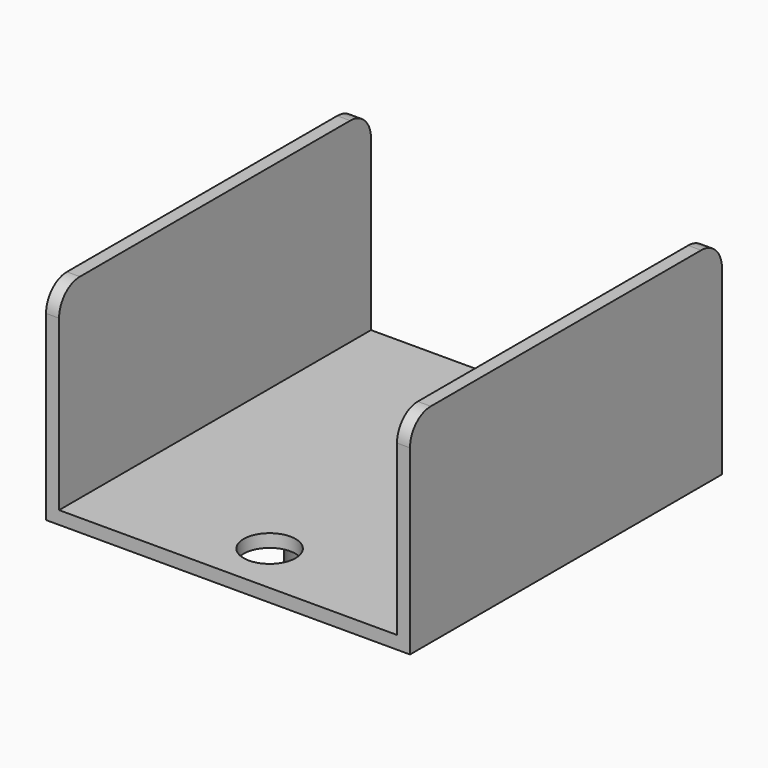
from build123d import *

# Parameters (mm, degrees)
F1_DEPTH = 30
F2_R     = 2.5
F3_DEPTH = 3
F4_R     = 6
F4_R_2   = 2.5
F5_DEPTH = 4
F6_R     = 2
F7_D     = 4
F7_DEPTH = 15
F7_TIP   = 1.2017212381


with BuildPart() as f1:
    # F0 (on Front) → F1 (new body)
    with BuildSketch(Plane.XZ):
        Polygon((0, 1), (0, 0), (28, 0), (28, 1), (28, 16), (27, 16), (27, 1), (1, 1), (1, 16), (0, 16), align=None)
    extrude(amount=-F1_DEPTH)

    # F2 (on face) → F3 (join)
    with BuildSketch(Plane.XY.offset(1)):
        with Locations((14, 15)):
            Circle(F2_R)
    extrude(amount=-F3_DEPTH)

    # F4 (on face) → F5 (join)
    with BuildSketch(Plane(origin=(0, 0, -2), x_dir=(1, 0, 0), z_dir=(0, 0, -1))):
        with Locations((14, -15)):
            Circle(F4_R)
        with Locations((14, -15)):
            Circle(F4_R_2, mode=Mode.SUBTRACT)
        with Locations((14, -15)):
            Circle(F4_R_2)
    extrude(amount=F5_DEPTH)

    # F6
    f6_edges = [f1.edges().sort_by_distance(p)[0] for p in [
        (27.5, 0, 16),
        (27.5, 30, 16),
        (0.5, 30, 16),
        (0.5, 0, 16),
    ]]
    fillet(f6_edges, radius=F6_R)

    # F7
    with Locations(Plane.XY.offset(1)):
        with Locations((14, 4), (14, 26)):
            Hole(F7_D / 2, depth=F7_DEPTH)
            with Locations((0, 0, -(F7_DEPTH + F7_TIP / 2))):  # 118° drill point
                Cone(0, F7_D / 2, F7_TIP, mode=Mode.SUBTRACT)


solid = f1.part
